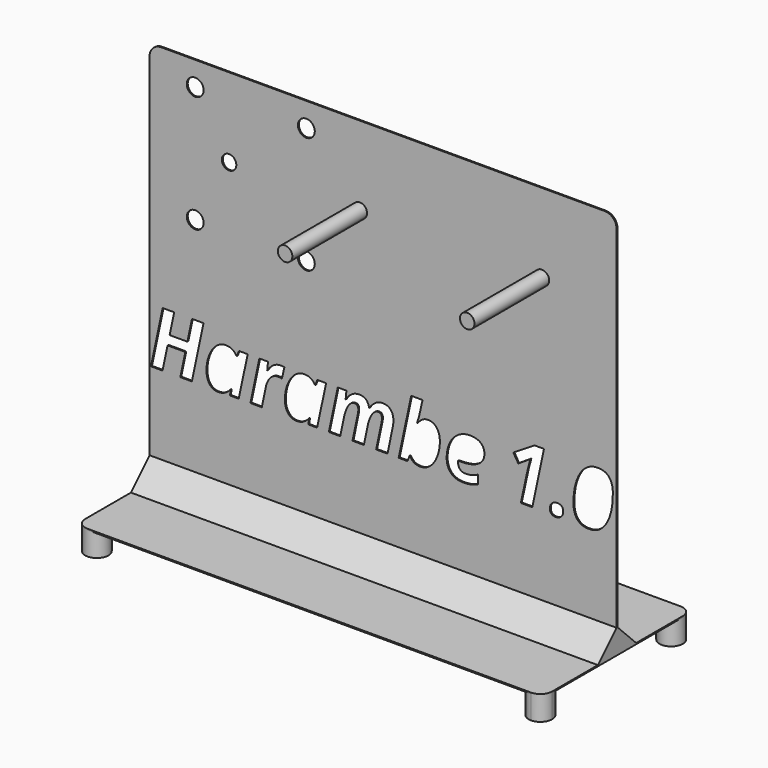
from build123d import *

# Parameters (mm, degrees)
F0_R     = 3.937
F1_DEPTH = 0.635
F2_D     = 9.1694
F3_R     = 3.937
F4_DEPTH = 50.8
F6_DEPTH = 0.635
F8_DEPTH = 12.7
F9_SIZE  = 12.7


# Not quite as in the source:
# - a feature names something its author has since deleted; it is built from what else it names


with BuildPart() as f1:
    # F0 (on Front) → F1 (new body)
    with BuildSketch(Plane.XZ):
        with BuildLine():
            Line((0, 76.598051393), (0, 6.35))
            Line((0, 6.35), (0, -120.8449261427))
            Line((0, -120.8449261427), (0, -127.1949261427))
            Line((0, -127.1949261427), (6.35, -127.1949261427))
            Line((6.35, -127.1949261427), (247.65, -127.1949261427))
            Line((247.65, -127.1949261427), (254, -127.1949261427))
            Line((254, -127.1949261427), (254, -120.8449261427))
            Line((254, -120.8449261427), (254, 6.35))
            Line((254, 6.35), (254, 76.598051393))
            ThreePointArc((254, 76.598051393), (252.1401280605, 81.0881794536), (247.65, 82.948051393))
            Line((247.65, 82.948051393), (6.35, 82.948051393))
            ThreePointArc((6.35, 82.948051393), (1.8598719395, 81.0881794536), (0, 76.598051393))
        make_face()
        Polygon((29.319182166, -41.6570965657), (22.9772223603, -71.6533847153), (16.7009143123, -71.6533847153), (19.4451577894, -58.7068580725), (9.7877842135, -58.7068580725), (7.0369755607, -71.6533847153), (0.7803630401, -71.6533847153), (7.1157576701, -41.6570965657), (13.3986308938, -41.6570965657), (10.9104292723, -53.4153263919), (20.5743680239, -53.4153263919), (23.0560044697, -41.6570965657), align=None, mode=Mode.SUBTRACT)
        with BuildLine():
            add(Edge.make_bspline(
                [(43.9857848639, -68.6793600859), (41.234976211, -72.0669907896), (37.4403046088, -72.0669907896)],
                knots=[0, 0, 0, 1, 1, 1], degree=2))
            add(Edge.make_bspline(
                [(37.4403046088, -72.0669907896), (34.4203237489, -72.0669907896), (32.6871173424, -69.8807872541)],
                knots=[0, 0, 0, 1, 1, 1], degree=2))
            add(Edge.make_bspline(
                [(32.6871173424, -69.8807872541), (30.9539109359, -67.6945837185), (30.9539109359, -63.7554782491)],
                knots=[0, 0, 0, 1, 1, 1], degree=2))
            add(Edge.make_bspline(
                [(30.9539109359, -63.7554782491), (30.9539109359, -59.6916344398), (32.4310754869, -56.0085708259)],
                knots=[0, 0, 0, 1, 1, 1], degree=2))
            add(Edge.make_bspline(
                [(32.4310754869, -56.0085708259), (33.9082400379, -52.325507212), (36.3110943743, -50.3067156589)],
                knots=[0, 0, 0, 1, 1, 1], degree=2))
            add(Edge.make_bspline(
                [(36.3110943743, -50.3067156589), (38.7139487106, -48.2879241059), (41.5829305275, -48.2879241059)],
                knots=[0, 0, 0, 1, 1, 1], degree=2))
            add(Edge.make_bspline(
                [(41.5829305275, -48.2879241059), (43.5721787896, -48.2879241059), (45.0198000496, -49.1479621333)],
                knots=[0, 0, 0, 1, 1, 1], degree=2))
            add(Edge.make_bspline(
                [(45.0198000496, -49.1479621333), (46.4674213096, -50.0080001608), (47.268372755, -51.6492941064)],
                knots=[0, 0, 0, 1, 1, 1], degree=2))
            Line((47.268372755, -51.6492941064), (47.4325021496, -51.6492941064))
            Line((47.4325021496, -51.6492941064), (48.6011034389, -48.7146605317))
            Line((48.6011034389, -48.7146605317), (53.3608558811, -48.7146605317))
            Line((53.3608558811, -48.7146605317), (48.476365099, -71.6533847153))
            Line((48.476365099, -71.6533847153), (43.7756992388, -71.6533847153))
            Line((43.7756992388, -71.6533847153), (44.0645669732, -68.6793600859))
            Line((44.0645669732, -68.6793600859), (43.9857848639, -68.6793600859))
        make_face(mode=Mode.SUBTRACT)
        with BuildLine():
            add(Edge.make_bspline(
                [(64.1080486368, -52.9623292629), (67.1280294967, -48.2879241059), (71.3494375248, -48.2879241059)],
                knots=[0, 0, 0, 1, 1, 1], degree=2))
            add(Edge.make_bspline(
                [(71.3494375248, -48.2879241059), (72.5639950445, -48.2879241059), (73.3189902595, -48.5111400825)],
                knots=[0, 0, 0, 1, 1, 1], degree=2))
            Line((73.3189902595, -48.5111400825), (71.9665640483, -54.4591893413))
            add(Edge.make_bspline(
                [(71.9665640483, -54.4591893413), (71.040874263, -54.1309305522), (69.9182292042, -54.1309305522)],
                knots=[0, 0, 0, 1, 1, 1], degree=2))
            add(Edge.make_bspline(
                [(69.9182292042, -54.1309305522), (67.5350703952, -54.1309305522), (65.7394948187, -56.0085708259)],
                knots=[0, 0, 0, 1, 1, 1], degree=2))
            add(Edge.make_bspline(
                [(65.7394948187, -56.0085708259), (63.9439192423, -57.8862110997), (63.1889240273, -61.3920149675)],
                knots=[0, 0, 0, 1, 1, 1], degree=2))
            Line((63.1889240273, -61.3920149675), (61.0092856675, -71.6533847153))
            Line((61.0092856675, -71.6533847153), (54.8380204321, -71.6533847153))
            Line((54.8380204321, -71.6533847153), (59.6962505111, -48.7146605317))
            Line((59.6962505111, -48.7146605317), (64.4166118986, -48.7146605317))
            Line((64.4166118986, -48.7146605317), (63.983310297, -52.9623292629))
            Line((63.983310297, -52.9623292629), (64.1080486368, -52.9623292629))
        make_face(mode=Mode.SUBTRACT)
        with BuildLine():
            add(Edge.make_bspline(
                [(86.6397319219, -68.6793600859), (83.8889232691, -72.0669907896), (80.0942516669, -72.0669907896)],
                knots=[0, 0, 0, 1, 1, 1], degree=2))
            add(Edge.make_bspline(
                [(80.0942516669, -72.0669907896), (77.074270807, -72.0669907896), (75.3410644005, -69.8807872541)],
                knots=[0, 0, 0, 1, 1, 1], degree=2))
            add(Edge.make_bspline(
                [(75.3410644005, -69.8807872541), (73.6078579939, -67.6945837185), (73.6078579939, -63.7554782491)],
                knots=[0, 0, 0, 1, 1, 1], degree=2))
            add(Edge.make_bspline(
                [(73.6078579939, -63.7554782491), (73.6078579939, -59.6916344398), (75.085022545, -56.0085708259)],
                knots=[0, 0, 0, 1, 1, 1], degree=2))
            add(Edge.make_bspline(
                [(75.085022545, -56.0085708259), (76.562187096, -52.325507212), (78.9650414323, -50.3067156589)],
                knots=[0, 0, 0, 1, 1, 1], degree=2))
            add(Edge.make_bspline(
                [(78.9650414323, -50.3067156589), (81.3678957687, -48.2879241059), (84.2368775856, -48.2879241059)],
                knots=[0, 0, 0, 1, 1, 1], degree=2))
            add(Edge.make_bspline(
                [(84.2368775856, -48.2879241059), (86.2261258476, -48.2879241059), (87.6737471077, -49.1479621333)],
                knots=[0, 0, 0, 1, 1, 1], degree=2))
            add(Edge.make_bspline(
                [(87.6737471077, -49.1479621333), (89.1213683677, -50.0080001608), (89.9223198131, -51.6492941064)],
                knots=[0, 0, 0, 1, 1, 1], degree=2))
            Line((89.9223198131, -51.6492941064), (90.0864492077, -51.6492941064))
            Line((90.0864492077, -51.6492941064), (91.2550504969, -48.7146605317))
            Line((91.2550504969, -48.7146605317), (96.0148029392, -48.7146605317))
            Line((96.0148029392, -48.7146605317), (91.1303121571, -71.6533847153))
            Line((91.1303121571, -71.6533847153), (86.4296462969, -71.6533847153))
            Line((86.4296462969, -71.6533847153), (86.7185140313, -68.6793600859))
            Line((86.7185140313, -68.6793600859), (86.6397319219, -68.6793600859))
        make_face(mode=Mode.SUBTRACT)
        with BuildLine():
            add(Edge.make_bspline(
                [(106.7619956949, -52.9623292629), (109.7557158517, -48.2879241059), (114.0493408133, -48.2879241059)],
                knots=[0, 0, 0, 1, 1, 1], degree=2))
            add(Edge.make_bspline(
                [(114.0493408133, -48.2879241059), (118.5399210485, -48.2879241059), (119.4196546033, -52.9623292629)],
                knots=[0, 0, 0, 1, 1, 1], degree=2))
            Line((119.4196546033, -52.9623292629), (119.5443929432, -52.9623292629))
            add(Edge.make_bspline(
                [(119.5443929432, -52.9623292629), (120.9427753848, -50.7039087938), (122.8401111859, -49.4959164498)],
                knots=[0, 0, 0, 1, 1, 1], degree=2))
            add(Edge.make_bspline(
                [(122.8401111859, -49.4959164498), (124.737446987, -48.2879241059), (126.8908246436, -48.2879241059)],
                knots=[0, 0, 0, 1, 1, 1], degree=2))
            add(Edge.make_bspline(
                [(126.8908246436, -48.2879241059), (129.6810243512, -48.2879241059), (131.1483411385, -50.0309782761)],
                knots=[0, 0, 0, 1, 1, 1], degree=2))
            add(Edge.make_bspline(
                [(131.1483411385, -50.0309782761), (132.6156579259, -51.7740324463), (132.6156579259, -54.8924909429)],
                knots=[0, 0, 0, 1, 1, 1], degree=2))
            add(Edge.make_bspline(
                [(132.6156579259, -54.8924909429), (132.6156579259, -56.4484376033), (132.1429652695, -58.5821197326)],
                knots=[0, 0, 0, 1, 1, 1], degree=2))
            Line((132.1429652695, -58.5821197326), (129.4118521441, -71.6533847153))
            Line((129.4118521441, -71.6533847153), (123.2405869087, -71.6533847153))
            Line((123.2405869087, -71.6533847153), (126.0701776709, -58.2538609435))
            add(Edge.make_bspline(
                [(126.0701776709, -58.2538609435), (126.39843646, -56.8620436776), (126.39843646, -55.8116155525)],
                knots=[0, 0, 0, 1, 1, 1], degree=2))
            add(Edge.make_bspline(
                [(126.39843646, -55.8116155525), (126.39843646, -53.290588052), (124.3894926706, -53.290588052)],
                knots=[0, 0, 0, 1, 1, 1], degree=2))
            add(Edge.make_bspline(
                [(124.3894926706, -53.290588052), (122.4987220452, -53.290588052), (120.9690360879, -55.5883995759)],
                knots=[0, 0, 0, 1, 1, 1], degree=2))
            add(Edge.make_bspline(
                [(120.9690360879, -55.5883995759), (119.4393501307, -57.8862110997), (118.5399210485, -62.1141843035)],
                knots=[0, 0, 0, 1, 1, 1], degree=2))
            Line((118.5399210485, -62.1141843035), (116.5703683138, -71.6533847153))
            Line((116.5703683138, -71.6533847153), (110.3925379025, -71.6533847153))
            Line((110.3925379025, -71.6533847153), (113.2024331374, -58.2538609435))
            add(Edge.make_bspline(
                [(113.2024331374, -58.2538609435), (113.5306919265, -56.8620436776), (113.5306919265, -55.8116155525)],
                knots=[0, 0, 0, 1, 1, 1], degree=2))
            add(Edge.make_bspline(
                [(113.5306919265, -55.8116155525), (113.5306919265, -53.290588052), (111.5217481371, -53.290588052)],
                knots=[0, 0, 0, 1, 1, 1], degree=2))
            add(Edge.make_bspline(
                [(111.5217481371, -53.290588052), (109.6375426876, -53.290588052), (108.0980089666, -55.6310732184)],
                knots=[0, 0, 0, 1, 1, 1], degree=2))
            add(Edge.make_bspline(
                [(108.0980089666, -55.6310732184), (106.5584752456, -57.9715583849), (105.6787416908, -62.1535753582)],
                knots=[0, 0, 0, 1, 1, 1], degree=2))
            Line((105.6787416908, -62.1535753582), (103.6632327256, -71.6533847153))
            Line((103.6632327256, -71.6533847153), (97.4919674902, -71.6533847153))
            Line((97.4919674902, -71.6533847153), (102.3501975691, -48.7146605317))
            Line((102.3501975691, -48.7146605317), (107.0705589567, -48.7146605317))
            Line((107.0705589567, -48.7146605317), (106.637257355, -52.9623292629))
            Line((106.637257355, -52.9623292629), (106.7619956949, -52.9623292629))
        make_face(mode=Mode.SUBTRACT)
        with BuildLine():
            add(Edge.make_bspline(
                [(148.5460569618, -49.0265063814), (149.868939882, -48.2879241059), (151.4314517182, -48.2879241059)],
                knots=[0, 0, 0, 1, 1, 1], degree=2))
            add(Edge.make_bspline(
                [(151.4314517182, -48.2879241059), (154.4251718749, -48.2879241059), (156.1583782815, -50.5036709324)],
                knots=[0, 0, 0, 1, 1, 1], degree=2))
            add(Edge.make_bspline(
                [(156.1583782815, -50.5036709324), (157.891584688, -52.719417759), (157.891584688, -56.6125669979)],
                knots=[0, 0, 0, 1, 1, 1], degree=2))
            add(Edge.make_bspline(
                [(157.891584688, -56.6125669979), (157.891584688, -60.5122814126), (156.4964848343, -64.152671384)],
                knots=[0, 0, 0, 1, 1, 1], degree=2))
            add(Edge.make_bspline(
                [(156.4964848343, -64.152671384), (155.1013849805, -67.7930613553), (152.6591395895, -69.9300260724)],
                knots=[0, 0, 0, 1, 1, 1], degree=2))
            add(Edge.make_bspline(
                [(152.6591395895, -69.9300260724), (150.2168941984, -72.0669907896), (147.2625650963, -72.0669907896)],
                knots=[0, 0, 0, 1, 1, 1], degree=2))
            add(Edge.make_bspline(
                [(147.2625650963, -72.0669907896), (143.2840685722, -72.0669907896), (141.6033835719, -68.7187511406)],
                knots=[0, 0, 0, 1, 1, 1], degree=2))
            Line((141.6033835719, -68.7187511406), (141.4392541774, -68.7187511406))
            Line((141.4392541774, -68.7187511406), (140.2509573608, -71.6533847153))
            Line((140.2509573608, -71.6533847153), (135.5109004459, -71.6533847153))
            Line((135.5109004459, -71.6533847153), (142.2795966775, -39.7269348856))
            Line((142.2795966775, -39.7269348856), (148.4574270887, -39.7269348856))
            Line((148.4574270887, -39.7269348856), (147.183782987, -45.6355930898))
            add(Edge.make_bspline(
                [(147.183782987, -45.6355930898), (146.3434404868, -49.3711781099), (145.4571417562, -51.7740324463)],
                knots=[0, 0, 0, 1, 1, 1], degree=2))
            Line((145.4571417562, -51.7740324463), (145.6212711508, -51.7740324463))
            add(Edge.make_bspline(
                [(145.6212711508, -51.7740324463), (147.2231740417, -49.7650886569), (148.5460569618, -49.0265063814)],
                knots=[0, 0, 0, 1, 1, 1], degree=2))
        make_face(mode=Mode.SUBTRACT)
        with BuildLine():
            add(Edge.make_bspline(
                [(178.6703660392, -70.3009585042), (175.1448666441, -72.0669907896), (170.6739819363, -72.0669907896)],
                knots=[0, 0, 0, 1, 1, 1], degree=2))
            add(Edge.make_bspline(
                [(170.6739819363, -72.0669907896), (166.3606614473, -72.0669907896), (163.9807852262, -69.7462011505)],
                knots=[0, 0, 0, 1, 1, 1], degree=2))
            add(Edge.make_bspline(
                [(163.9807852262, -69.7462011505), (161.600909005, -67.4254115115), (161.600909005, -63.1974383076)],
                knots=[0, 0, 0, 1, 1, 1], degree=2))
            add(Edge.make_bspline(
                [(161.600909005, -63.1974383076), (161.600909005, -58.9563347522), (163.2947243569, -55.4570960602)],
                knots=[0, 0, 0, 1, 1, 1], degree=2))
            add(Edge.make_bspline(
                [(163.2947243569, -55.4570960602), (164.9885397088, -51.9578573682), (167.8804996409, -50.122890737)],
                knots=[0, 0, 0, 1, 1, 1], degree=2))
            add(Edge.make_bspline(
                [(167.8804996409, -50.122890737), (170.772459573, -48.2879241059), (174.422697308, -48.2879241059)],
                knots=[0, 0, 0, 1, 1, 1], degree=2))
            add(Edge.make_bspline(
                [(174.422697308, -48.2879241059), (178.0598046915, -48.2879241059), (180.0884440082, -49.9587613425)],
                knots=[0, 0, 0, 1, 1, 1], degree=2))
            add(Edge.make_bspline(
                [(180.0884440082, -49.9587613425), (182.117083325, -51.6295985791), (182.117083325, -54.5445366265)],
                knots=[0, 0, 0, 1, 1, 1], degree=2))
            add(Edge.make_bspline(
                [(182.117083325, -54.5445366265), (182.117083325, -58.3785992834), (178.6933441545, -60.4597600064)],
                knots=[0, 0, 0, 1, 1, 1], degree=2))
            add(Edge.make_bspline(
                [(178.6933441545, -60.4597600064), (175.2696049839, -62.5409207294), (168.9079496508, -62.5409207294)],
                knots=[0, 0, 0, 1, 1, 1], degree=2))
            Line((168.9079496508, -62.5409207294), (167.8575215256, -62.5409207294))
            Line((167.8575215256, -62.5409207294), (167.818130471, -62.974222331))
            Line((167.818130471, -62.974222331), (167.818130471, -63.3878284053))
            add(Edge.make_bspline(
                [(167.818130471, -63.3878284053), (167.818130471, -65.2523383275), (168.8751237719, -66.3290271558)],
                knots=[0, 0, 0, 1, 1, 1], degree=2))
            add(Edge.make_bspline(
                [(168.8751237719, -66.3290271558), (169.9321170729, -67.4057159841), (171.9016698076, -67.4057159841)],
                knots=[0, 0, 0, 1, 1, 1], degree=2))
            add(Edge.make_bspline(
                [(171.9016698076, -67.4057159841), (173.6873976204, -67.4057159841), (175.1448666441, -67.0150880251)],
                knots=[0, 0, 0, 1, 1, 1], degree=2))
            add(Edge.make_bspline(
                [(175.1448666441, -67.0150880251), (176.6023356678, -66.624460066), (178.6703660392, -65.6396836987)],
                knots=[0, 0, 0, 1, 1, 1], degree=2))
            Line((178.6703660392, -65.6396836987), (178.6703660392, -70.3009585042))
        make_face(mode=Mode.SUBTRACT)
        with BuildLine():
            add(Edge.make_bspline(
                [(218.5800696203, -71.4367339145), (217.7397271201, -70.668608348), (217.7397271201, -69.2964866094)],
                knots=[0, 0, 0, 1, 1, 1], degree=2))
            add(Edge.make_bspline(
                [(217.7397271201, -69.2964866094), (217.7397271201, -67.4451070388), (218.8393940637, -66.3388749195)],
                knots=[0, 0, 0, 1, 1, 1], degree=2))
            add(Edge.make_bspline(
                [(218.8393940637, -66.3388749195), (219.9390610072, -65.2326428002), (221.9283092693, -65.2326428002)],
                knots=[0, 0, 0, 1, 1, 1], degree=2))
            add(Edge.make_bspline(
                [(221.9283092693, -65.2326428002), (223.3201265351, -65.2326428002), (224.1604690353, -66.0106161304)],
                knots=[0, 0, 0, 1, 1, 1], degree=2))
            add(Edge.make_bspline(
                [(224.1604690353, -66.0106161304), (225.0008115354, -66.7885894606), (225.0008115354, -68.2066674296)],
                knots=[0, 0, 0, 1, 1, 1], degree=2))
            add(Edge.make_bspline(
                [(225.0008115354, -68.2066674296), (225.0008115354, -69.9923952424), (223.8748838887, -71.0986273617)],
                knots=[0, 0, 0, 1, 1, 1], degree=2))
            add(Edge.make_bspline(
                [(223.8748838887, -71.0986273617), (222.7489562421, -72.204859481), (220.9238373746, -72.204859481)],
                knots=[0, 0, 0, 1, 1, 1], degree=2))
            add(Edge.make_bspline(
                [(220.9238373746, -72.204859481), (219.4204121204, -72.204859481), (218.5800696203, -71.4367339145)],
                knots=[0, 0, 0, 1, 1, 1], degree=2))
        make_face(mode=Mode.SUBTRACT)
        with BuildLine():
            Line((214.5424865141, -41.6570965657), (208.2005267083, -71.6533847153))
            Line((208.2005267083, -71.6533847153), (201.9439141877, -71.6533847153))
            Line((201.9439141877, -71.6533847153), (205.6335429774, -54.6430142632))
            add(Edge.make_bspline(
                [(205.6335429774, -54.6430142632), (206.3557123135, -51.5245557666), (207.1960548136, -48.7540515864)],
                knots=[0, 0, 0, 1, 1, 1], degree=2))
            add(Edge.make_bspline(
                [(207.1960548136, -48.7540515864), (207.0122298917, -48.918180981), (205.9355410634, -49.7191324264)],
                knots=[0, 0, 0, 1, 1, 1], degree=2))
            add(Edge.make_bspline(
                [(205.9355410634, -49.7191324264), (204.8588522351, -50.5200838719), (200.5455317461, -53.2118059426)],
                knots=[0, 0, 0, 1, 1, 1], degree=2))
            Line((200.5455317461, -53.2118059426), (197.8209837964, -48.8000078169))
            Line((197.8209837964, -48.8000078169), (209.4347797554, -41.6570965657))
            Line((209.4347797554, -41.6570965657), (214.5424865141, -41.6570965657))
        make_face(mode=Mode.SUBTRACT)
        with BuildLine():
            add(Edge.make_bspline(
                [(243.7969098003, -41.1844039093), (251.983684001, -41.1844039093), (251.983684001, -50.8877337157)],
                knots=[0, 0, 0, 1, 1, 1], degree=2))
            add(Edge.make_bspline(
                [(251.983684001, -50.8877337157), (251.983684001, -60.53197694), (248.5271189515, -66.2994838648)],
                knots=[0, 0, 0, 1, 1, 1], degree=2))
            add(Edge.make_bspline(
                [(248.5271189515, -66.2994838648), (245.0705539021, -72.0669907896), (238.8336369089, -72.0669907896)],
                knots=[0, 0, 0, 1, 1, 1], degree=2))
            add(Edge.make_bspline(
                [(238.8336369089, -72.0669907896), (234.7697930996, -72.0669907896), (232.6656542613, -69.5623762286)],
                knots=[0, 0, 0, 1, 1, 1], degree=2))
            add(Edge.make_bspline(
                [(232.6656542613, -69.5623762286), (230.5615154231, -67.0577616677), (230.5615154231, -62.0747932488)],
                knots=[0, 0, 0, 1, 1, 1], degree=2))
            add(Edge.make_bspline(
                [(230.5615154231, -62.0747932488), (230.5615154231, -55.975744947), (232.284874066, -51.0518631102)],
                knots=[0, 0, 0, 1, 1, 1], degree=2))
            add(Edge.make_bspline(
                [(232.284874066, -51.0518631102), (234.0082327088, -46.1279812735), (236.9625618109, -43.6561925914)],
                knots=[0, 0, 0, 1, 1, 1], degree=2))
            add(Edge.make_bspline(
                [(236.9625618109, -43.6561925914), (239.916890913, -41.1844039093), (243.7969098003, -41.1844039093)],
                knots=[0, 0, 0, 1, 1, 1], degree=2))
        make_face(mode=Mode.SUBTRACT)
        with Locations((43.2311252226, 39.878)):
            Circle(F0_R, mode=Mode.SUBTRACT)
    extrude(amount=F1_DEPTH)

    # F2 (through all)
    with Locations(Plane(origin=(0, 0, 0), x_dir=(1, 0, 0), z_dir=(0, 1, 0))):
        with Locations((24.8161252226, -69.85), (85.2681252226, -69.85), (85.2681252226, -6.35), (24.8161252226, -6.35)):
            Hole(F2_D / 2)

    # F3 (on face) → F4 (join)
    with BuildSketch(Plane.XZ.offset(0.635)):
        with Locations((114.3511252226, 39.878)):
            Circle(F3_R)
        with Locations((213.4111252226, 39.878)):
            Circle(F3_R)
    extrude(amount=F4_DEPTH)

    # F5 (on face) → F6 (join)
    with BuildSketch(Plane(origin=(0, 0, -127.1949261427), x_dir=(1, 0, 0), z_dir=(0, 0, -1))):
        with BuildLine():
            Line((0, 44.45), (0, -44.45))
            ThreePointArc((0, -44.45), (1.8598719395, -48.9401280605), (6.35, -50.8))
            Line((6.35, -50.8), (247.65, -50.8))
            ThreePointArc((247.65, -50.8), (252.1401280605, -48.9401280605), (254, -44.45))
            Line((254, -44.45), (254, 44.45))
            ThreePointArc((254, 44.45), (252.1401280605, 48.9401280605), (247.65, 50.8))
            Line((247.65, 50.8), (6.35, 50.8))
            ThreePointArc((6.35, 50.8), (1.8598719395, 48.9401280605), (0, 44.45))
        make_face()
    extrude(amount=F6_DEPTH)

    # F7 (on face) → F8 (join)
    with BuildSketch(Plane(origin=(0, 0, -127.8299261427), x_dir=(1, 0, 0), z_dir=(0, 0, -1))):
        with BuildLine():
            ThreePointArc((254, 44.45), (252.1401280605, 48.9401280605), (247.65, 50.8))
            ThreePointArc((247.65, 50.8), (243.1598719395, 39.9598719395), (254, 44.45))
        make_face()
        with BuildLine():
            ThreePointArc((247.65, -50.8), (252.1401280605, -48.9401280605), (254, -44.45))
            ThreePointArc((254, -44.45), (243.1598719395, -39.9598719395), (247.65, -50.8))
        make_face()
        with BuildLine():
            ThreePointArc((12.7, -44.45), (6.35, -38.1), (0, -44.45))
            ThreePointArc((0, -44.45), (1.8598719395, -48.9401280605), (6.35, -50.8))
            ThreePointArc((6.35, -50.8), (10.8401280605, -48.9401280605), (12.7, -44.45))
        make_face()
        with BuildLine():
            ThreePointArc((0, 44.45), (6.35, 38.1), (12.7, 44.45))
            ThreePointArc((12.7, 44.45), (10.8401280605, 48.9401280605), (6.35, 50.8))
            ThreePointArc((6.35, 50.8), (1.8598719395, 48.9401280605), (0, 44.45))
        make_face()
    extrude(amount=F8_DEPTH)

    # F9
    f9_edges = [f1.edges().sort_by_distance(p)[0] for p in [
        (127, -0.635, -127.194926),
        (127, 0, -127.194926),
    ]]
    chamfer(f9_edges, length=F9_SIZE)


solid = f1.part
